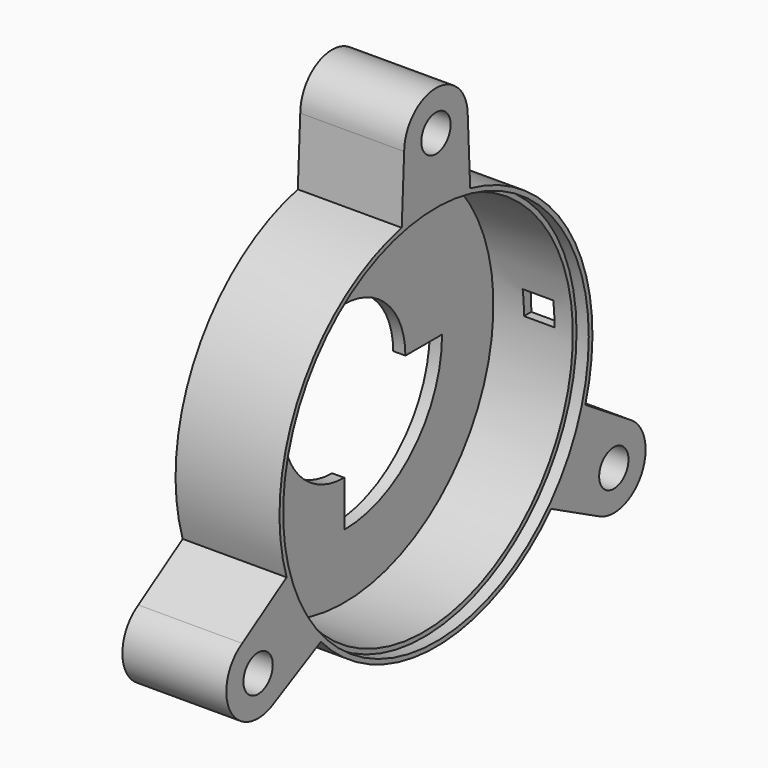
from build123d import *

# Parameters (mm, degrees)
F0_R            = 30.5
F0_R_2          = 9.5
F1_DEPTH        = 2
F2_R            = 32
F2_R_2          = 30.5
F3_DEPTH        = 17
F4_R            = 3
F5_DEPTH        = 17
F5_COPIES_COUNT = 3
F6_R            = 31.25
F7_DEPTH        = 2
F8_W            = 5
F8_H            = 4
F9_DEPTH        = 43.1
F10_R           = 5
F11_DEPTH       = 10
F13_DEPTH       = 25


# Not quite as in the source:
# - a pattern or mirror of a feature is missing from the dataset's text; its kind, count and spacing are read off the source's solid


with BuildPart() as f1:
    # F0 (on Right) → F1 (new body)
    with BuildSketch(Plane.YZ):
        Circle(F0_R)
        Circle(F0_R_2, mode=Mode.SUBTRACT)
    extrude(amount=F1_DEPTH)

    # F2 (on face) → F3 (join)
    with BuildSketch(Plane(origin=(0, 0, 0), x_dir=(0, -1, 0), z_dir=(-1, 0, 0))):
        Circle(F2_R)
        Circle(F2_R_2, mode=Mode.SUBTRACT)
    extrude(amount=-F3_DEPTH)

    # F4 (on face) → F5 (join)
    with BuildSketch(Plane.YZ.offset(17)):
        with BuildLine():
            ThreePointArc((-6.5, 42), (0, 35.5), (6.5, 42))
            ThreePointArc((6.5, 42), (0, 48.5), (-6.5, 42))
        make_face()
        with Locations((0, 42)):
            Circle(F4_R, mode=Mode.SUBTRACT)
        with BuildLine():
            Line((7, 31.224989992), (6.5, 42))
            ThreePointArc((6.5, 42), (0, 35.5), (-6.5, 42))
            Line((-6.5, 42), (-7, 31.224989992))
            ThreePointArc((-7, 31.224989992), (0, 32), (7, 31.224989992))
        make_face()
    f5 = extrude(amount=-F5_DEPTH)

    # F5_copies: F5 ×3 about axis
    f5_copies_axis = Axis((0, 0, 0), (1, 0, 0))
    for i in range(1, F5_COPIES_COUNT):
        add(f5.rotate(f5_copies_axis, i * 360 / F5_COPIES_COUNT))

    # F6 (on face) → F7 (cut)
    with BuildSketch(Plane.YZ.offset(17)):
        Circle(F6_R)
    extrude(amount=-F7_DEPTH, mode=Mode.SUBTRACT)

    # F8 (on Front) → F9 (cut)
    with BuildSketch(Plane.XZ):
        with Locations((9.5, 2)):
            Rectangle(F8_W, F8_H)
    extrude(amount=-F9_DEPTH, mode=Mode.SUBTRACT)

    # F10 (on face) → F11 (cut)
    with BuildSketch(Plane(origin=(0, 0, 0), x_dir=(0, -1, 0), z_dir=(-1, 0, 0))):
        with Locations((-36.3730669589, -21)):
            Circle(F10_R)
        with Locations((0, 42)):
            Circle(F10_R)
        with Locations((36.3730669589, -21)):
            Circle(F10_R)
    extrude(amount=-F11_DEPTH, mode=Mode.SUBTRACT)

    # F12 (on face) → F13 (cut)
    with BuildSketch(Plane(origin=(0, 0, 0), x_dir=(0, -1, 0), z_dir=(-1, 0, 0))):
        with BuildLine():
            Line((-12.5, 0), (-20, 0))
            ThreePointArc((-20, 0), (-14.1421356237, -14.1421356237), (0, -20))
            Line((0, -20), (0, -12.5))
            ThreePointArc((0, -12.5), (8.8388347648, -8.8388347648), (12.5, 0))
            Line((12.5, 0), (20, 0))
            ThreePointArc((20, 0), (14.1421356237, 14.1421356237), (0, 20))
            Line((0, 20), (0, 12.5))
            ThreePointArc((0, 12.5), (-8.8388347648, 8.8388347648), (-12.5, 0))
        make_face()
    extrude(amount=-F13_DEPTH, mode=Mode.SUBTRACT)


solid = f1.part
